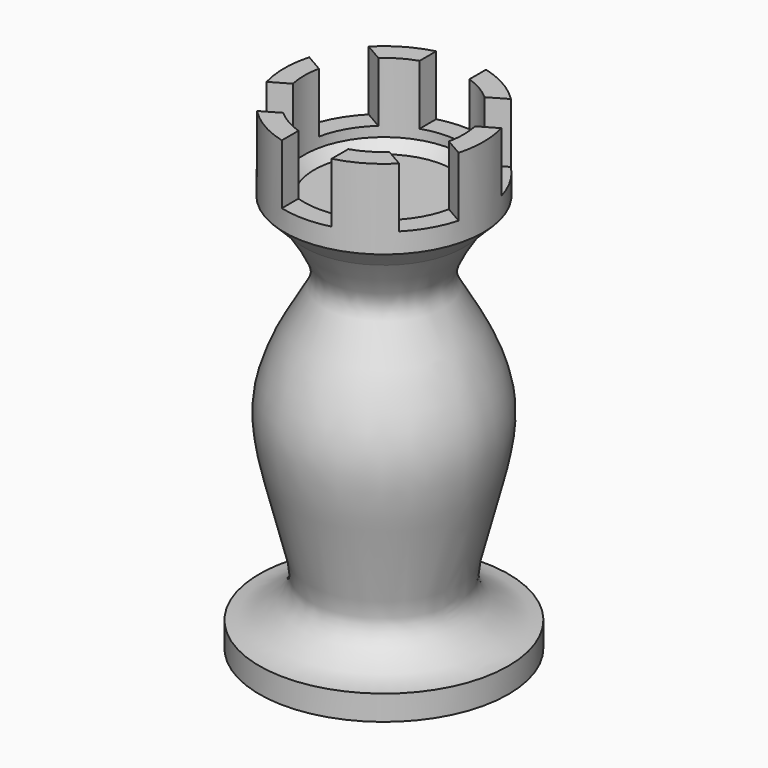
from build123d import *

# Parameters (mm, degrees)
F0_W            = 12.5
F0_H            = 2.5
F2_W            = 5
F2_H            = 30
F3_DEPTH        = 6
F3_COPIES_COUNT = 3
F3_COPIES_ANGLE = 120
F4_SIZE         = 1


# Not quite as in the source:
# - a pattern or mirror of a feature is missing from the dataset's text; its kind, count and spacing are read off the source's solid


with BuildPart() as f1:
    # F0 (on Front) → F1 (revolve)
    with BuildSketch(Plane.XZ):
        with BuildLine():
            Line((0, 38), (0, 2.5))
            Line((0, 2.5), (12.5, 2.5))
            add(Edge.make_bspline(
                [(8, 38), (7.0207852122, 36.4938667138), (5.4043126084, 34.0070254969), (5.9600054984, 31.8314336156), (8.1990620491, 28.5626744432), (10.3907797529, 23.474773004), (10.4814127916, 17.8992218413), (7.2195549415, 7.8955797317), (7.4012690721, 4.6378342418), (10.7296475451, 2.5), (12.5, 2.5)],
                knots=[0, 0, 0, 0, 0.1240829897, 0.2038473168, 0.3165719642, 0.4493670123, 0.5879210693, 0.7717537445, 0.8711203486, 1, 1, 1, 1], degree=3))
            Line((8, 38), (0, 38))
        make_face()
        Polygon((0, 40), (0, 38), (8, 38), (10, 40), (10, 48), (8, 48), (8, 40), align=None)
        with Locations((6.25, 1.25)):
            Rectangle(F0_W, F0_H)
    revolve(axis=Axis((0, 0, 24), (0, 0, 1)))

    # F2 (on face) → F3 (cut)
    with BuildSketch(Plane.XY.offset(48)):
        Rectangle(F2_W, F2_H)
    f3 = extrude(amount=-F3_DEPTH, mode=Mode.SUBTRACT)

    # F3_copies: F3 ×3 about axis
    f3_copies_axis = Axis((0, 0, 0), (0, 0, 1))
    for i in range(1, F3_COPIES_COUNT):
        add(f3.rotate(f3_copies_axis, i * F3_COPIES_ANGLE / (F3_COPIES_COUNT - 1)), mode=Mode.SUBTRACT)

    # F4
    f4_edges = [f1.edges().sort_by_distance(p)[0] for p in [
        (-8, 0, 40),
    ]]
    chamfer(f4_edges, length=F4_SIZE)


solid = f1.part
